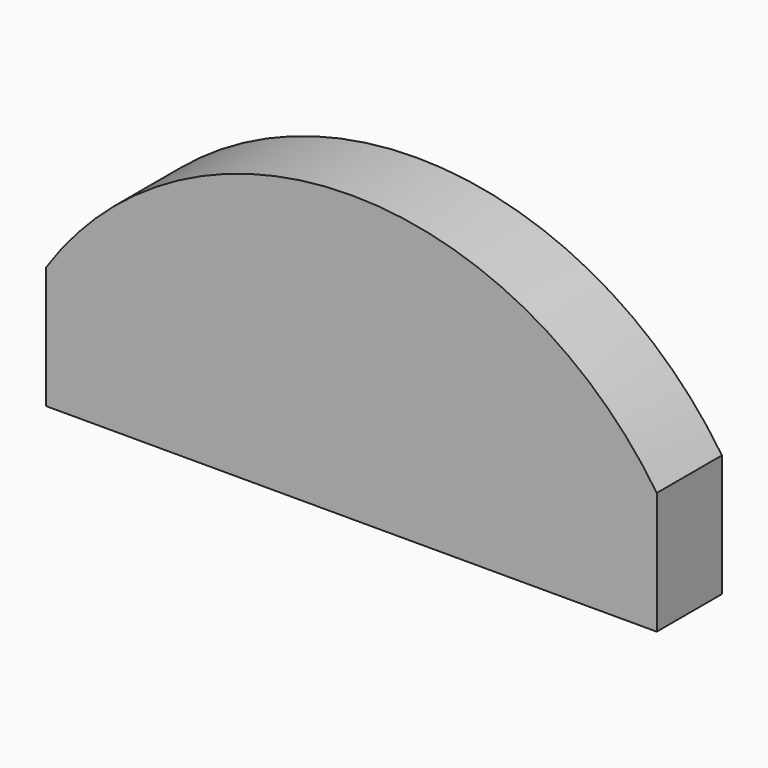
from build123d import *

# Parameters (mm, degrees)
F1_DEPTH = 20


# Not quite as in the source:
# - a feature names something its author has since deleted; it is built from what else it names


with BuildPart() as f1:
    # F0 (on Front) → F1 (new body)
    with BuildSketch(Plane.XZ):
        with BuildLine():
            ThreePointArc((84.7183704376, 29.7274781391), (9.7183704376, 69.7274781391), (-65.2816295624, 29.7274781391))
            Line((-65.2816295624, 29.7274781391), (-65.2816295624, -0.2725218609))
            Line((-65.2816295624, -0.2725218609), (84.7183704376, -0.2725218609))
            Line((84.7183704376, -0.2725218609), (84.7183704376, 29.7274781391))
        make_face()
    extrude(amount=F1_DEPTH)


solid = f1.part
